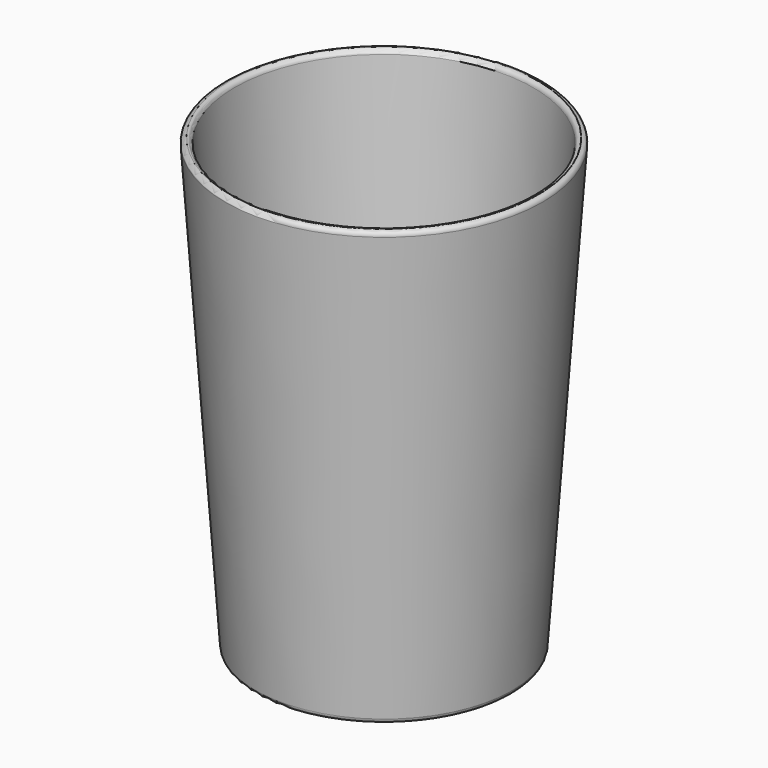
from build123d import *

# Parameters (mm, degrees)
F2_R = 0.99999


# Not quite as in the source:
# - a fillet or chamfer is up to 0.001 mm smaller than in the source, because OpenCascade refuses the exact size


with BuildPart() as f1:
    # F0 (on Front) → F1 (revolve)
    with BuildSketch(Plane.XZ):
        Polygon((-31.9951162038, 79.5454481112), (-34, 79.5454481112), (-27.2870260534, -16.4545518888), (0, -16.4545518888), (0, -14.4545518888), (-25.4219958811, -14.4545518888), align=None)
    revolve(axis=Axis((0, 0, -15.4545518888), (0, 0, 1)))

    # F2 (radius 1 in the source; OpenCascade refuses exactly that, so slightly less here)
    f2_edges = [f1.edges().sort_by_distance(p)[0] for p in [
        (27.287026, 0, -16.454552),
        (34, 0, 79.545448),
        (31.995116, 0, 79.545448),
    ]]
    fillet(f2_edges, radius=F2_R)


solid = f1.part
